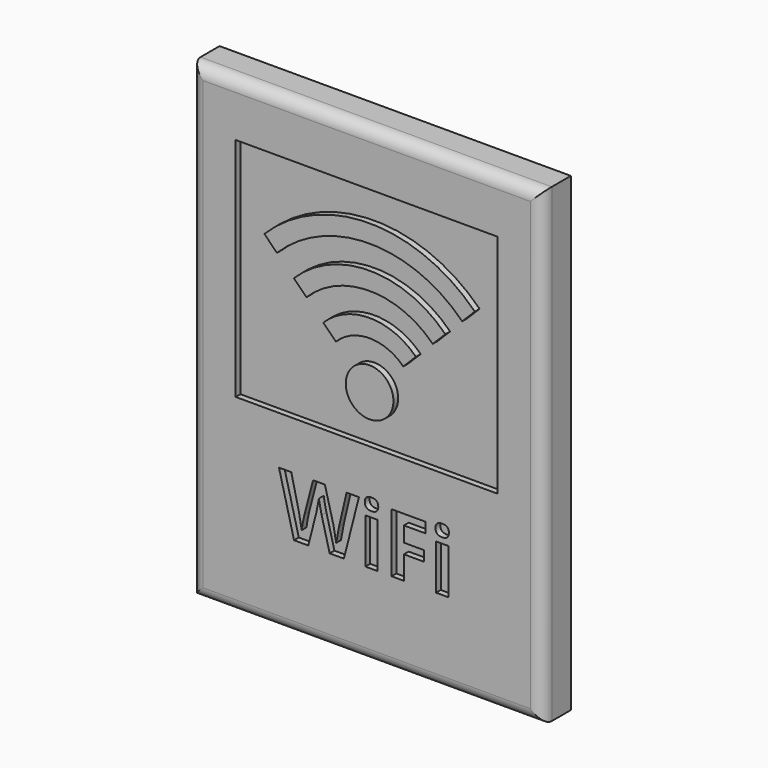
from build123d import *

# Parameters (mm, degrees)
F0_W         = 29.5
F0_H         = 39.5
F1_DEPTH     = 3
F2_R         = 1
F3_W         = 22
F3_H         = 19
F3_R         = 2
F4_DEPTH     = 0.5
F5_TEXT_SIZE = 6.9444444444
F6_DEPTH     = 0.5
F7_W         = 25
F7_H         = 35
F8_DEPTH     = 1


# Not quite as in the source:
# - Text() gives the source's letters only with a copy of the font that has no kerning and outlines rounded to 1/6400 em; it was checked with that copy


with BuildPart() as f1:
    # F0 (on Front) → F1 (new body)
    with BuildSketch(Plane.XZ):
        with Locations((14.75, 19.75)):
            Rectangle(F0_W, F0_H)
    extrude(amount=F1_DEPTH)

    # F2
    f2_edges = [f1.edges().sort_by_distance(p)[0] for p in [
        (29.5, -3, 19.75),
        (14.75, -3, 0),
        (0, -3, 19.75),
        (14.75, -3, 39.5),
    ]]
    fillet(f2_edges, radius=F2_R)

    # F3 (on face) → F4 (cut)
    with BuildSketch(Plane.XZ.offset(3)):
        with Locations((14.75, 25.5)):
            Rectangle(F3_W, F3_H)
        with Locations((15, 20)):
            Circle(F3_R, mode=Mode.SUBTRACT)
        with BuildLine():
            ThreePointArc((17.8284271247, 22.8284271247), (15, 24), (12.1715728753, 22.8284271247))
            Line((12.1715728753, 22.8284271247), (11.1109127035, 23.8890872965))
            ThreePointArc((11.1109127035, 23.8890872965), (15, 25.5), (18.8890872965, 23.8890872965))
            Line((18.8890872965, 23.8890872965), (17.8284271247, 22.8284271247))
        make_face(mode=Mode.SUBTRACT)
        with BuildLine():
            ThreePointArc((20.3033008589, 25.3033008589), (15, 27.5), (9.6966991411, 25.3033008589))
            Line((9.6966991411, 25.3033008589), (8.6360389693, 26.3639610307))
            ThreePointArc((8.6360389693, 26.3639610307), (15, 29), (21.3639610307, 26.3639610307))
            Line((21.3639610307, 26.3639610307), (20.3033008589, 25.3033008589))
        make_face(mode=Mode.SUBTRACT)
        with BuildLine():
            ThreePointArc((22.7781745931, 27.7781745931), (15, 31), (7.2218254069, 27.7781745931))
            Line((7.2218254069, 27.7781745931), (6.1611652352, 28.8388347648))
            ThreePointArc((6.1611652352, 28.8388347648), (15, 32.5), (23.8388347648, 28.8388347648))
            Line((23.8388347648, 28.8388347648), (22.7781745931, 27.7781745931))
        make_face(mode=Mode.SUBTRACT)
    extrude(amount=-F4_DEPTH, mode=Mode.SUBTRACT)

    # F5 (on face) → F6 (cut)
    with BuildSketch(Plane.XZ.offset(3)):
        with Locations((7.3899739583, 7)):
            Text('WiFi', F5_TEXT_SIZE, font='Open Sans', font_style=FontStyle.BOLD, text_align=(TextAlign.LEFT, TextAlign.BOTTOM))
    extrude(amount=-F6_DEPTH, mode=Mode.SUBTRACT)

    # F7 (on face) → F8 (cut)
    with BuildSketch(Plane(origin=(0, 0, 0), x_dir=(-1, 0, 0), z_dir=(0, 1, 0))):
        with Locations((-14.75, 20.0430153636)):
            Rectangle(F7_W, F7_H)
    extrude(amount=-F8_DEPTH, mode=Mode.SUBTRACT)


solid = f1.part
